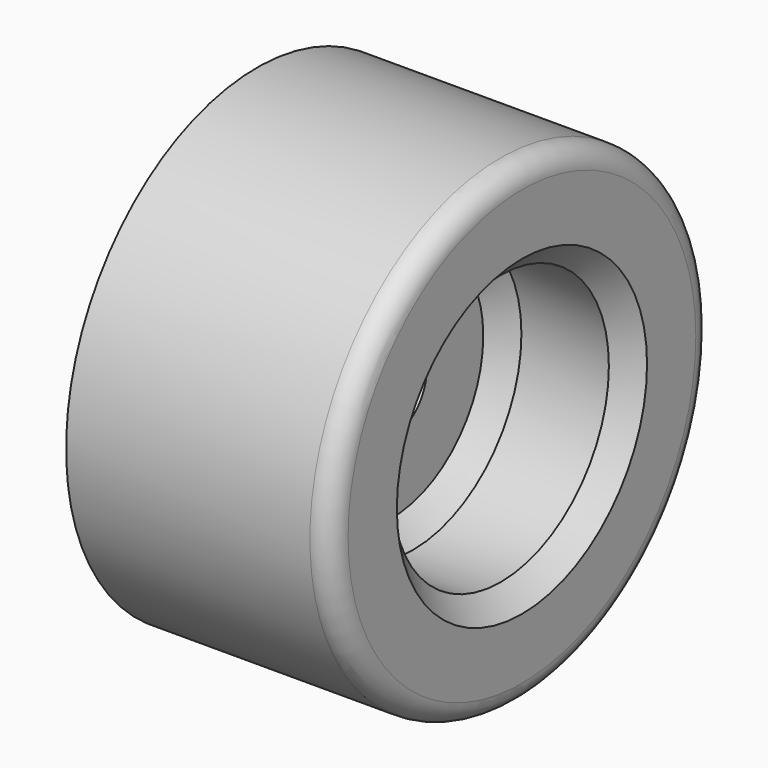
from build123d import *

# Parameters (mm, degrees)
F0_R     = 225
F0_R_2   = 127.5080178576
F1_DEPTH = 125
F0_R_3   = 21
F2_DEPTH = 2.5
F3_R     = 20


# Not quite as in the source:
# - a fillet or chamfer that OpenCascade refuses, or shapes differently, is made with other operations: its cross-section is extruded or revolved along the edge and cut away or added


with BuildPart() as f1:
    # F0 (on Right) → F1 (new body, symmetric)
    with BuildSketch(Plane.YZ):
        Circle(F0_R)
        Circle(F0_R_2, mode=Mode.SUBTRACT)
    extrude(amount=F1_DEPTH, both=True)

    # F0 (on Right) → F2 (join, symmetric)
    with BuildSketch(Plane.YZ):
        Circle(F0_R_2)
        Circle(F0_R_3, mode=Mode.SUBTRACT)
    extrude(amount=F2_DEPTH, both=True)

    # F3
    f3_edges = [f1.edges().sort_by_distance(p)[0] for p in [
        (125, -225, 0),
    ]]
    fillet(f3_edges, radius=F3_R)

    # F4: chamfer of 20 on 5 edges, made by hand

    # F4_s1 → F4_t2 (revolve)
    with BuildSketch(Plane.XY):
        Polygon((-22.5, 127.5080178576), (-2.5, 107.5080178576), (-2.5, 127.5080178576), align=None)
    revolve(axis=Axis((-2.5, 0, 0), (1, 0, 0)))

    # F4_s3 → F4_t4 (revolve)
    with BuildSketch(Plane.XY):
        Polygon((22.5, 127.5080178576), (2.5, 107.5080178576), (2.5, 127.5080178576), align=None)
    revolve(axis=Axis((2.5, 0, 0), (1, 0, 0)))

    # F4_s5 → F4_t6 (revolve, cut)
    with BuildSketch(Plane.XY):
        Polygon((-125, 147.5080178576), (-105, 127.5080178576), (-125, 127.5080178576), align=None)
    revolve(axis=Axis((-125, 0, 0), (1, 0, 0)), mode=Mode.SUBTRACT)

    # F4_s7 → F4_t8 (revolve, cut)
    with BuildSketch(Plane.XY):
        Polygon((125, 147.5080178576), (105, 127.5080178576), (125, 127.5080178576), align=None)
    revolve(axis=Axis((125, 0, 0), (1, 0, 0)), mode=Mode.SUBTRACT)

    # F4_s9 → F4_t10 (revolve, cut)
    with BuildSketch(Plane.XY):
        Polygon((2.5, 41), (-17.5, 21), (2.5, 21), align=None)
    revolve(axis=Axis((2.5, 0, 0), (1, 0, 0)), mode=Mode.SUBTRACT)


solid = f1.part
